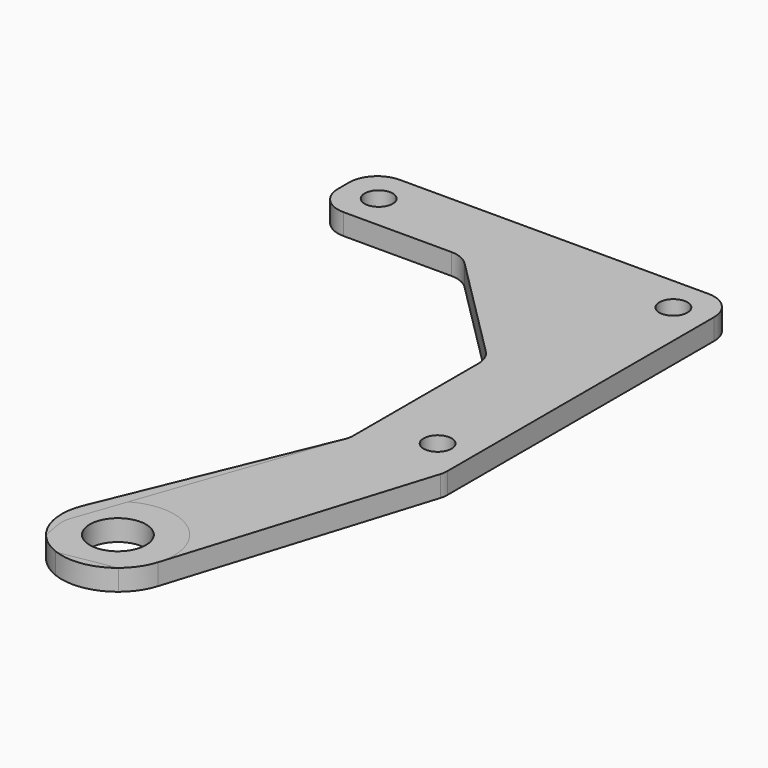
from build123d import *
from build123d import SkipClean  # not in build123d's __all__

# Parameters (mm, degrees)
F0_W     = 10.5
F0_H     = 5
F0_R     = 1
F0_R_2   = 2
F1_DEPTH = 1.5
F2_R     = 2
F4_DEPTH = 1.5
F3_R     = 1
F5_DEPTH = 1.5


with BuildPart() as f1:
    # F0 (on Top) → F1 (new body)
    with BuildSketch(Plane.XY):
        with Locations((-5.25, 23.5)):
            Rectangle(F0_W, F0_H)
        with Locations((-8, 23.5)):
            Circle(F0_R, mode=Mode.SUBTRACT)
        Polygon((8.75, 21), (0, 21), (8.75, 12.25), align=None)
        Polygon((8.75, 2.5), (8.75, 0), (15.5, 0), (15.5, 26), (0, 26), (0, 21), (8.75, 21), (8.75, 12.25), align=None)
        with Locations((13, 2.5)):
            Circle(F0_R, mode=Mode.SUBTRACT)
        with Locations((13, 23.5)):
            Circle(F0_R, mode=Mode.SUBTRACT)
        Polygon((15.5, 0), (8.75, 0), (2.5261364178, -17.8039236821), (3.1339050396, -21.2507508176), (10.0275593107, -20.035213574), align=None)
        with Locations((5.9729635533, -17.1961550602)):
            Circle(F0_R_2, mode=Mode.SUBTRACT)
    extrude(amount=F1_DEPTH)

    # F2
    f2_edges = [f1.edges().sort_by_distance(p)[0] for p in [
        (3.133905, -21.250751, 0.75),
        (2.526136, -17.803924, 0.75),
        (10.027559, -20.035214, 0.75),
        (0, 21, 0.75),
        (8.75, 12.25, 0.75),
        (8.75, 0, 0.75),
        (15.5, 0, 0.75),
        (-10.5, 21, 0.75),
        (-10.5, 26, 0.75),
        (15.5, 26, 0.75),
    ]]
    fillet(f2_edges, radius=F2_R)

    # F3 (on face) → F4 (cut, through all)
    with BuildSketch(Plane.XY.offset(1.5)):
        with BuildLine():
            Line((15.4293248166, -0.2587497013), (9.7925199679, -18.3840055542))
            ThreePointArc((9.7925199679, -18.3840055542), (9.2828500145, -19.4421852503), (8.4878041885, -20.3067139457))
            Line((8.4878041885, -20.3067139457), (8.7794635144, -20.2552865373))
            ThreePointArc((8.7794635144, -20.2552865373), (9.7797768114, -19.7634897702), (10.3614919757, -18.8126489739))
            Line((10.3614919757, -18.8126489739), (15.4293248166, -0.2587497013))
        make_face()
        with BuildLine():
            ThreePointArc((2.9760281468, -19.8453772421), (3.6090713176, -20.5721430448), (4.5085212955, -20.9184404971))
            ThreePointArc((4.5085212955, -20.9184404971), (3.6786578079, -20.4727632374), (2.9760281468, -19.8453772421))
        make_face()
    extrude(amount=-F4_DEPTH, mode=Mode.SUBTRACT)

    # F3 (on face) → F5 (join)
    with BuildSketch(Plane.XY.offset(1.5)):
        with BuildLine():
            ThreePointArc((2.2760890833, -15.6686999373), (2.9532568393, -14.5729182502), (3.9435858611, -13.7491815787))
            Line((3.9435858611, -13.7491815787), (8.6379648829, -0.3204865672))
            ThreePointArc((8.6379648829, -0.3204865672), (8.6665084457, -0.2323302993), (8.6909380974, -0.1429465499))
            Line((8.6909380974, -0.1429465499), (2.2760890833, -15.6686999373))
        make_face()
        with BuildLine():
            Line((2.6984727346, -17.3109400888), (3.9435858611, -13.7491815787))
            ThreePointArc((3.9435858611, -13.7491815787), (2.9532568393, -14.5729182502), (2.2760890833, -15.6686999373))
            ThreePointArc((2.2760890833, -15.6686999373), (2.027975468, -17.8572670075), (2.9760281468, -19.8453772421))
            ThreePointArc((2.9760281468, -19.8453772421), (2.8602115576, -19.570341978), (2.7866086843, -19.2811353116))
            Line((2.7866086843, -19.2811353116), (2.6168221115, -18.3182278083))
            ThreePointArc((2.6168221115, -18.3182278083), (2.5929761176, -17.8093417002), (2.6984727346, -17.3109400888))
        make_face()
        with BuildLine():
            ThreePointArc((4.5085212955, -20.9184404971), (6.5807353289, -21.1497121256), (8.4878041885, -20.3067139457))
            Line((8.4878041885, -20.3067139457), (5.1035205457, -20.9034544623))
            ThreePointArc((5.1035205457, -20.9034544623), (4.8065815101, -20.9332048908), (4.5085212955, -20.9184404971))
        make_face()
        with BuildLine():
            ThreePointArc((9.9729635533, -17.1961550602), (9.927595373, -17.7968939144), (9.7925199679, -18.3840055542))
            Line((9.7925199679, -18.3840055542), (15.4293248166, -0.2587497013))
            ThreePointArc((15.4293248166, -0.2587497013), (15.4822524604, 0.0023801957), (15.5, 0.2682282413))
            Line((15.5, 0.2682282413), (15.5, 24))
            ThreePointArc((15.5, 24), (14.9142135624, 25.4142135624), (13.5, 26))
            Line((13.5, 26), (-8.5, 26))
            ThreePointArc((-8.5, 26), (-9.9142135624, 25.4142135624), (-10.5, 24))
            Line((-10.5, 24), (-10.5, 23))
            ThreePointArc((-10.5, 23), (-9.9142135624, 21.5857864376), (-8.5, 21))
            Line((-8.5, 21), (-0.8284271247, 21))
            ThreePointArc((-0.8284271247, 21), (-0.06306026, 20.847759065), (0.5857864376, 20.4142135624))
            Line((0.5857864376, 20.4142135624), (8.1642135624, 12.8357864376))
            ThreePointArc((8.1642135624, 12.8357864376), (8.597759065, 12.18693974), (8.75, 11.4215728753))
            Line((8.75, 11.4215728753), (8.75, 0.339504797))
            ThreePointArc((8.75, 0.339504797), (8.7351796134, 0.0964782499), (8.6909380974, -0.1429465499))
            ThreePointArc((8.6909380974, -0.1429465499), (8.6665084457, -0.2323302993), (8.6379648829, -0.3204865672))
            Line((8.6379648829, -0.3204865672), (3.9435858611, -13.7491815787))
            ThreePointArc((3.9435858611, -13.7491815787), (7.9582203668, -13.7235831914), (9.9729635533, -17.1961550602))
        make_face()
        with Locations((-8, 23.5)):
            Circle(F3_R, mode=Mode.SUBTRACT)
        with Locations((13, 2.5)):
            Circle(F3_R, mode=Mode.SUBTRACT)
        with Locations((13, 23.5)):
            Circle(F3_R, mode=Mode.SUBTRACT)
    with SkipClean():  # cleaning this boolean's faces spoils the solid; the shape is the same uncleaned
        extrude(amount=-F5_DEPTH)


solid = f1.part
